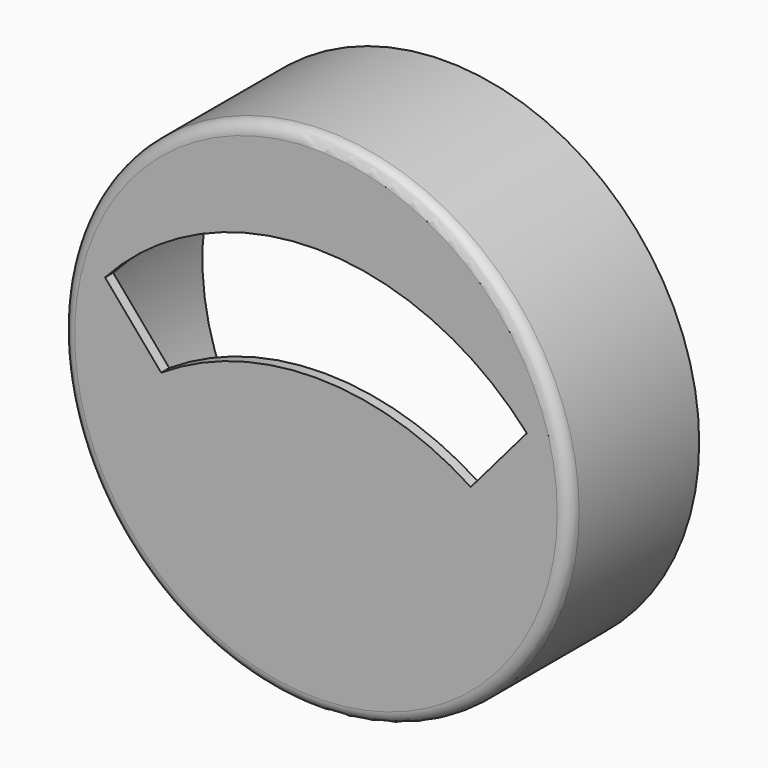
from build123d import *

# Parameters (mm, degrees)
F0_R             = 62.5
F1_DEPTH         = 40
F2_R             = 3
F3_T             = -2.5
F5_DEPTH         = 2.5
F6_R             = 2.5
F7_DEPTH         = 13
F8_R             = 1
F9_DEPTH         = 8
F12_DEPTH        = 1
F12_COPIES_COUNT = 3
F12_COPIES_ANGLE = 180
F15_DEPTH        = 1
F15_DEPTH_BACK   = 1
F15_COPIES_COUNT = 3
F15_COPIES_ANGLE = 180


# Not quite as in the source:
# - a pattern or mirror of a feature is missing from the dataset's text; its kind, count and spacing are read off the source's solid


with BuildPart() as f1:
    # F0 (on Front) → F1 (new body)
    with BuildSketch(Plane.XZ):
        Circle(F0_R)
    extrude(amount=F1_DEPTH)

    # F2
    f2_edges = [f1.edges().sort_by_distance(p)[0] for p in [
        (-62.5, -40, 0),
    ]]
    fillet(f2_edges, radius=F2_R)

    # F3
    f3_openings = [f1.faces().sort_by_distance(p)[0] for p in [
        (0, 0, 0),
    ]]
    offset(amount=F3_T, openings=f3_openings)

    # F4 (on face) → F5 (cut, through all)
    with BuildSketch(Plane.XZ.offset(40)):
        with BuildLine():
            ThreePointArc((52, 14.8614980554), (0, 38), (-52, 14.8614980554))
            Line((-52, 14.8614980554), (-38.1715582316, -1.3234958252))
            ThreePointArc((-38.1715582316, -1.3234958252), (0, 10), (38.1715582316, -1.3234958252))
            Line((38.1715582316, -1.3234958252), (52, 14.8614980554))
        make_face()
    extrude(amount=-F5_DEPTH, mode=Mode.SUBTRACT)

    # F6 (on face) → F7 (join)
    with BuildSketch(Plane(origin=(0, -37.5, 0), x_dir=(-1, 0, 0), z_dir=(0, 1, 0))):
        with Locations((-8.6170678389, -47.5194215546)):
            Circle(F6_R)
        with Locations((18.9575492455, -42.6572725799)):
            Circle(F6_R)
    extrude(amount=F7_DEPTH)

    # F8 (on face) → F9 (cut)
    with BuildSketch(Plane(origin=(0, -24.5, 0), x_dir=(-1, 0, 0), z_dir=(0, 1, 0))):
        with Locations((-8.6170678389, -47.5194215546)):
            Circle(F8_R)
        with Locations((18.9575492455, -42.6572725799)):
            Circle(F8_R)
    extrude(amount=-F9_DEPTH, mode=Mode.SUBTRACT)

    # F11 (on face) → F12 (join, symmetric)
    with BuildSketch(Plane(origin=(27.0393139988, 0, -15.6111552159), x_dir=(0, -1, 0), z_dir=(-0.8660254038, 0, 0.5))):
        Polygon((28.5, -34.84449232), (37.5, -34.84449232), (37.5, -28.84449232), align=None)
    f12 = extrude(amount=F12_DEPTH, both=True)

    # F12_copies: F12 ×3 about axis
    f12_copies_axis = Axis((8.617068, 0, -47.519422), (0, 1, 0))
    for i in range(1, F12_COPIES_COUNT):
        add(f12.rotate(f12_copies_axis, i * F12_COPIES_ANGLE / (F12_COPIES_COUNT - 1)))

    # F14 (on face) → F15 (join, two sides)
    with BuildSketch(Plane(origin=(-18.9575492455, 0, 0), x_dir=(0, -1, 0), z_dir=(-1, 0, 0))) as f15_sk:
        Polygon((28.5, -40.6572725799), (37.5, -40.6572725799), (37.5, -40.1572725799), (37.5, -34.6572725799), align=None)
    f15 = extrude(amount=F15_DEPTH) + extrude(f15_sk.sketch, amount=-F15_DEPTH_BACK)

    # F15_copies: F15 ×3 about axis
    f15_copies_axis = Axis((-18.957549, 0, -42.657273), (0, -1, 0))
    for i in range(1, F15_COPIES_COUNT):
        add(f15.rotate(f15_copies_axis, i * F15_COPIES_ANGLE / (F15_COPIES_COUNT - 1)))


solid = f1.part
